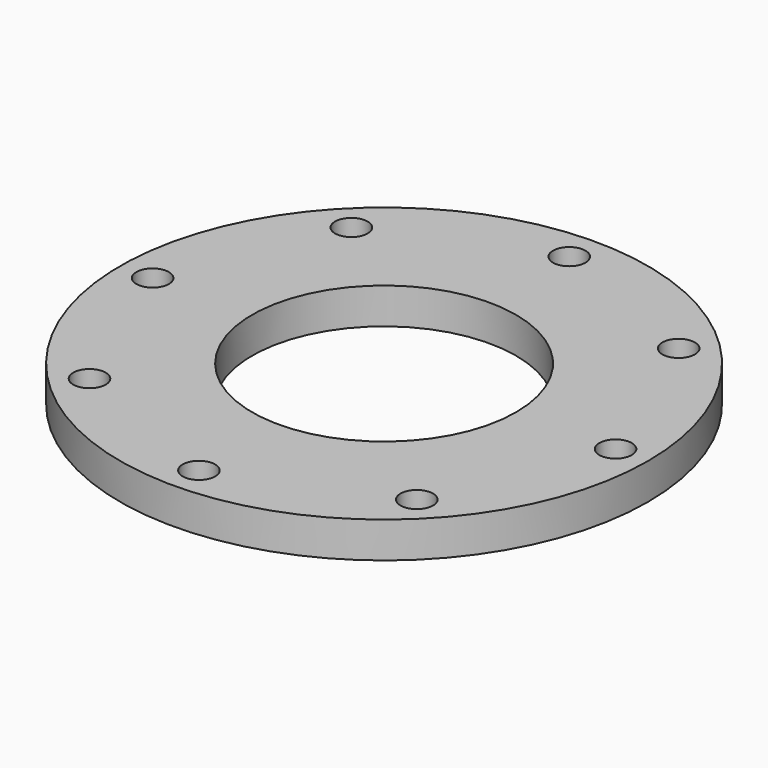
from build123d import *

# Parameters (mm, degrees)
F0_R            = 139.7
F1_DEPTH        = 19.05
F2_R            = 69.85
F3_DEPTH        = 19.051
F4_R            = 8.60044
F5_DEPTH        = 19.051
F5_COPIES_COUNT = 8


# Not quite as in the source:
# - a pattern or mirror of a feature is missing from the dataset's text; its kind, count and spacing are read off the source's solid


with BuildPart() as f1:
    # F0 (on Top) → F1 (new body)
    with BuildSketch(Plane.XY):
        Circle(F0_R)
    extrude(amount=F1_DEPTH)

    # F2 (on face) → F3 (cut, through all)
    with BuildSketch(Plane.XY.offset(19.05)):
        Circle(F2_R)
    extrude(amount=-F3_DEPTH, mode=Mode.SUBTRACT)

    # F4 (on face) → F5 (cut, through all)
    with BuildSketch(Plane.XY.offset(19.05)):
        with Locations((122.50039, 0)):
            Circle(F4_R)
    f5 = extrude(amount=-F5_DEPTH, mode=Mode.SUBTRACT)

    # F5_copies: F5 ×8 about axis
    f5_copies_axis = Axis((0, 0, 0), (0, 0, 1))
    for i in range(1, F5_COPIES_COUNT):
        add(f5.rotate(f5_copies_axis, i * 360 / F5_COPIES_COUNT), mode=Mode.SUBTRACT)


solid = f1.part
